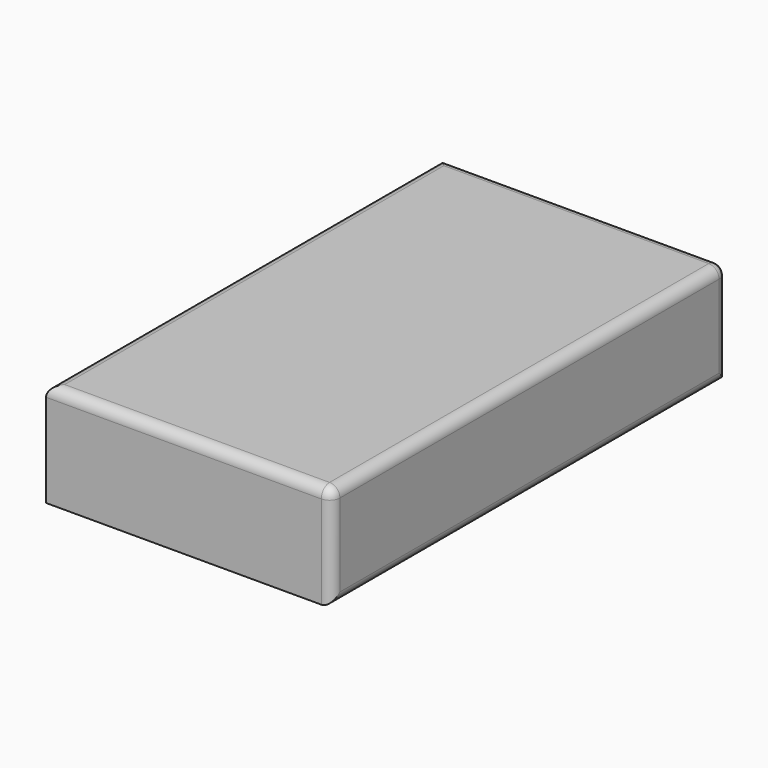
from build123d import *

# Parameters (mm, degrees)
F0_W     = 27.6158377528
F0_H     = 47.8320233524
F1_DEPTH = 10
F2_R     = 1


# Not quite as in the source:
# - the program builds the solid bodies; features that only make, move or delete a surface that nothing else refers to are left out


with BuildPart() as f1:
    # F0 (on Top) → F1 (new body)
    with BuildSketch(Plane.XY):
        with Locations((-22.0598205924, 4.9366392195)):
            Rectangle(F0_W, F0_H)
    extrude(amount=F1_DEPTH)

    # F2
    f2_edges = [f1.edges().sort_by_distance(p)[0] for p in [
        (-8.251902, -18.979372, 5),
        (-8.251902, 28.852651, 5),
        (-8.251902, 4.936639, 0),
        (-8.251902, 4.936639, 10),
        (-22.059821, 28.852651, 10),
        (-35.867739, 4.936639, 10),
        (-22.059821, -18.979372, 10),
    ]]
    fillet(f2_edges, radius=F2_R)


solid = f1.part
